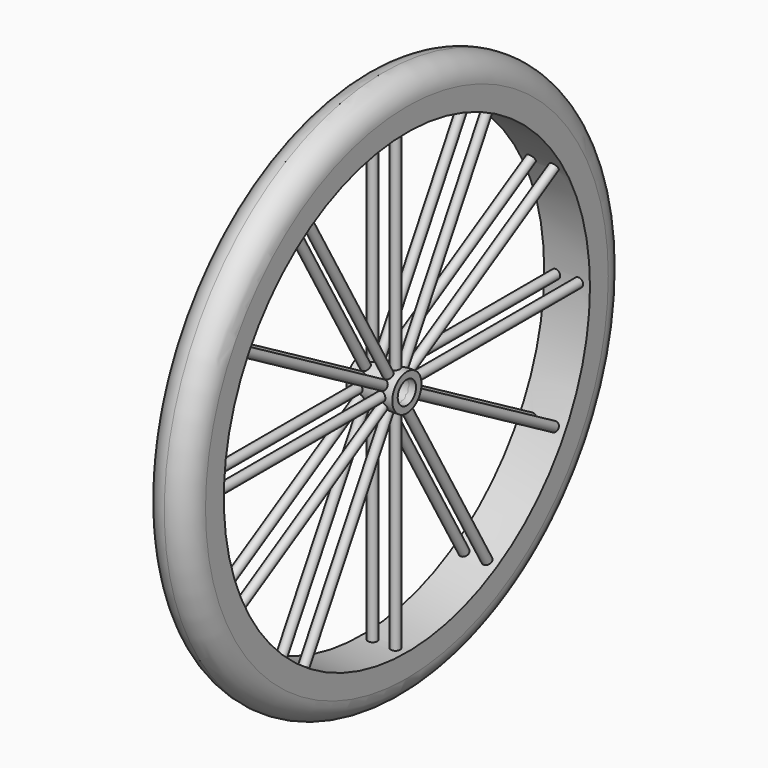
from build123d import *

# Parameters (mm, degrees)
F0_R     = 38.1
F0_R_2   = 31.75
F1_DEPTH = 6.35
F2_R     = 3.17499
F4_DEPTH = 33.02
F5_COUNT = 12
F5_ANGLE = 330
F6_R     = 1.5875
F7_DEPTH = 25.4
F8_R     = 2.54
F8_R_2   = 1.5875
F9_DEPTH = 6.35


# Not quite as in the source:
# - a fillet or chamfer is up to 0.001 mm smaller than in the source, because OpenCascade refuses the exact size


with BuildPart() as f1:
    # F0 (on Right) → F1 (new body)
    with BuildSketch(Plane.YZ):
        Circle(F0_R)
        Circle(F0_R_2, mode=Mode.SUBTRACT)
    extrude(amount=F1_DEPTH)

    # F2 (radius 3.175 in the source; OpenCascade refuses exactly that, so slightly less here)
    f2_edges = [f1.edges().sort_by_distance(p)[0] for p in [
        (6.35, -38.1, 0),
        (0, -38.1, 0),
    ]]
    fillet(f2_edges, radius=F2_R)



with BuildPart() as f4:
    # F3 (on Top) → F4 (new body)
    with BuildSketch(Plane.XY):
        with BuildLine():
            ThreePointArc((5.3975, 0), (4.7625, 0.635), (4.1275, 0))
            Line((4.1275, 0), (5.3975, 0))
        make_face()
        with BuildLine():
            Line((5.3975, 0), (4.1275, 0))
            ThreePointArc((4.1275, 0), (4.7625, -0.635), (5.3975, 0))
        make_face()
    extrude(amount=F4_DEPTH)


with BuildPart() as f4b:
    # F3 (on Top) → F4, piece 2 (new body)
    with BuildSketch(Plane.XY):
        with BuildLine():
            ThreePointArc((0.9525, 0), (1.5875, -0.635), (2.2225, 0))
            Line((2.2225, 0), (0.9525, 0))
        make_face()
        with BuildLine():
            Line((0.9525, 0), (2.2225, 0))
            ThreePointArc((2.2225, 0), (1.5875, 0.635), (0.9525, 0))
        make_face()
    extrude(amount=F4_DEPTH)


with BuildPart() as f1_1:
    add(f1.part)

    add(f4.part)  # F5 merges F4

    add(f4b.part)  # F5 merges F4b
    # F5: F4, F4b ×12 about axis
    f5_axis = Axis((6.35, 0, 0), (1, 0, 0))
    for i in range(1, F5_COUNT):
        add(f4.part.rotate(f5_axis, i * F5_ANGLE / (F5_COUNT - 1)))
        add(f4b.part.rotate(f5_axis, i * F5_ANGLE / (F5_COUNT - 1)))

    # F6 (on Right) → F7 (cut)
    with BuildSketch(Plane.YZ):
        Circle(F6_R)
    extrude(amount=F7_DEPTH, mode=Mode.SUBTRACT)

    # F8 (on Right) → F9 (join)
    with BuildSketch(Plane.YZ):
        Circle(F8_R)
        Circle(F8_R_2, mode=Mode.SUBTRACT)
    extrude(amount=F9_DEPTH)


solid = f1_1.part
